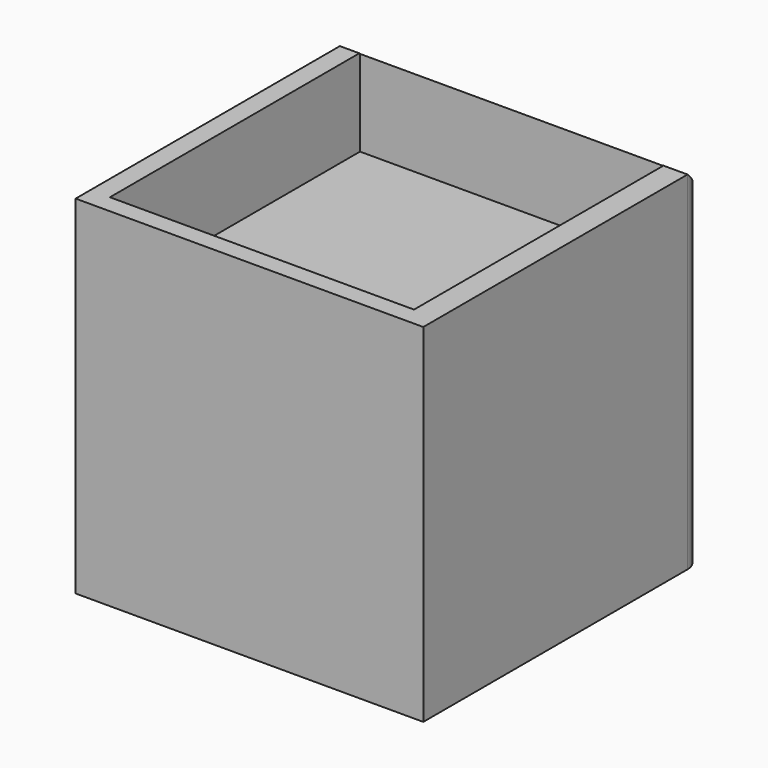
from build123d import *

# Parameters (mm, degrees)
F0_W        = 100
F0_H        = 100
F1_DEPTH    = 100
F2_W        = 87.4791443348
F2_H        = 89.9195559323
F3_DEPTH    = 25
F4_T1_DEPTH = 125.7168298797
F5_R        = 5


# Not quite as in the source:
# - a fillet or chamfer that OpenCascade refuses, or shapes differently, is made with other operations: its cross-section is extruded or revolved along the edge and cut away or added


with BuildPart() as f1:
    # F0 (on Top) → F1 (new body)
    with BuildSketch(Plane.XY):
        Rectangle(F0_W, F0_H)
    extrude(amount=F1_DEPTH)

    # F2 (on face) → F3 (cut)
    with BuildSketch(Plane.XY.offset(100)):
        with Locations((-0.6570331752, 0.2815853804)):
            Rectangle(F2_W, F2_H)
    extrude(amount=-F3_DEPTH, mode=Mode.SUBTRACT)

    # F4: chamfer of 5 on 1 edges, made by hand

    # F4_s2 → F4_t1 (cut)
    with BuildSketch(Plane.YZ.offset(-62.8584149398)):
        Polygon((50, 95), (45, 100), (50, 100), align=None)
    extrude(amount=F4_T1_DEPTH, mode=Mode.SUBTRACT)

    # F5
    f5_edges = [f1.edges().sort_by_distance(p)[0] for p in [
        (50, 50, 47.5),
    ]]
    fillet(f5_edges, radius=F5_R)


solid = f1.part
